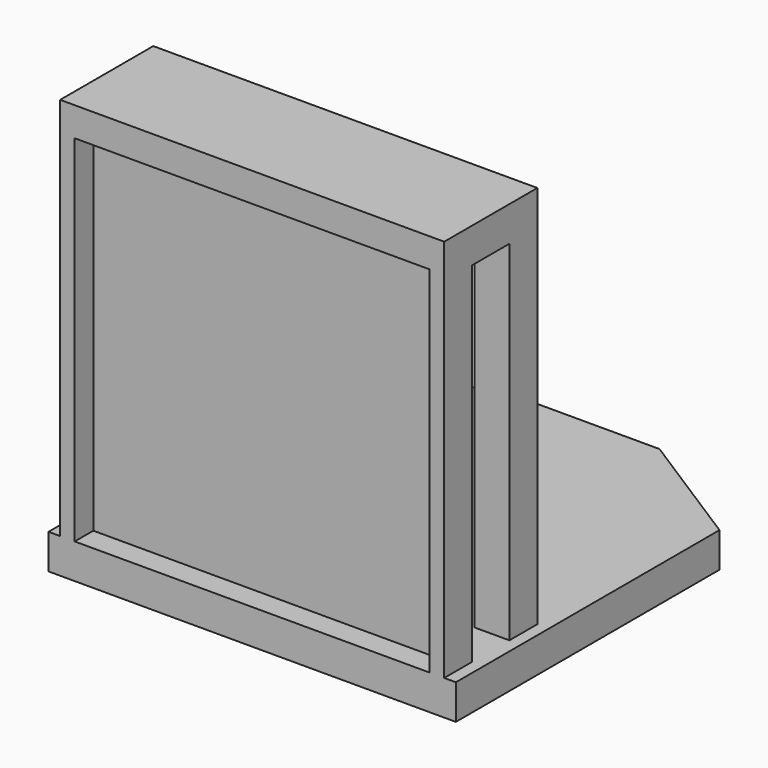
from build123d import *

# Parameters (mm, degrees)
F1_DEPTH = 3
F2_W     = 33
F2_H     = 3
F2_W_2   = 3
F3_DEPTH = 30
F4_W     = 33
F4_H     = 7
F4_H_2   = 3
F5_DEPTH = 3
F6_W     = 30.5
F6_H     = 30.5
F7_DEPTH = 2


# Not quite as in the source:
# - a feature names something its author has since deleted; it is built from what else it names


with BuildPart() as f1:
    # F0 (on Top) → F1 (new body)
    with BuildSketch(Plane.XY):
        Polygon((17.5, 10.8150299639), (7, 17.5), (-7, 17.5), (-17.5, 10.8150299639), (-17.5, -17.5), (17.5, -17.5), align=None)
    extrude(amount=F1_DEPTH)

    # F2 (on face) → F3 (join)
    with BuildSketch(Plane.XY.offset(3)):
        with Locations((0, -16)):
            Rectangle(F2_W, F2_H)
        with Locations((-15, -9)):
            Rectangle(F2_W_2, F2_H)
        with Locations((15, -9)):
            Rectangle(F2_W_2, F2_H)
    extrude(amount=F3_DEPTH)

    # F4 (on face) → F5 (join)
    with BuildSketch(Plane.XY.offset(33)):
        with Locations((0, -11)):
            Rectangle(F4_W, F4_H)
        with Locations((0, -16)):
            Rectangle(F4_W, F4_H_2)
    extrude(amount=F5_DEPTH)

    # F6 (on face) → F7 (cut)
    with BuildSketch(Plane.XZ.offset(17.5)):
        with Locations((0, 18.25)):
            Rectangle(F6_W, F6_H)
    extrude(amount=-F7_DEPTH, mode=Mode.SUBTRACT)


solid = f1.part
